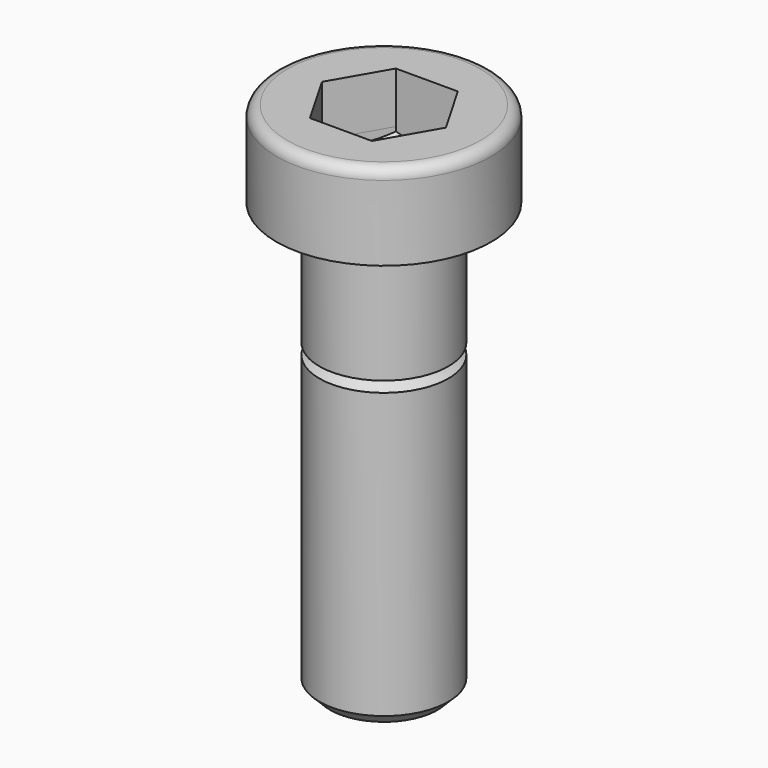
from build123d import *

# Parameters (mm, degrees)
F2_R     = 0.5
F3_SIZE  = 0.5
F5_DEPTH = 2.38


# Not quite as in the source:
# - a fillet or chamfer that OpenCascade refuses, or shapes differently, is made with other operations: its cross-section is extruded or revolved along the edge and cut away or added


with BuildPart() as f1:
    # F0 (on Front) → F1 (revolve)
    with BuildSketch(Plane.XZ):
        Polygon((-3, 0), (0, 0), (0, 18), (-1.5, 18.8660254038), (-1.5, 24), (-5, 24), (-5, 20), (-3, 20), (-3, 14.25), (-2.5, 14), (-3, 13.75), align=None)
    revolve(axis=Axis((0, 0, 18.332445994), (0, 0, 1)))

    # F2
    f2_edges = [f1.edges().sort_by_distance(p)[0] for p in [
        (5, 0, 24),
    ]]
    fillet(f2_edges, radius=F2_R)

    # F3
    f3_edges = [f1.edges().sort_by_distance(p)[0] for p in [
        (3, 0, 0),
    ]]
    chamfer(f3_edges, length=F3_SIZE)

    # F4 (on face) → F5 (cut)
    with BuildSketch(Plane.XY.offset(24)):
        Polygon((-1.443375673, -2.5), (1.443375673, -2.5), (2.8867513459, 0), (1.443375673, 2.5), (-1.443375673, 2.5), (-2.8867513459, 0), align=None)
    extrude(amount=-F5_DEPTH, mode=Mode.SUBTRACT)

    # F6: chamfer of 1 x 1.7320508076 on 1 edges, made by hand


with BuildPart() as f6_tool2:
    # F6_s3 → F6_t4 (revolve)
    with BuildSketch(Plane.XZ):
        Polygon((-3.2320508076, 21.62), (-1.5, 20.62), (-1.5, 21.62), align=None)
    revolve(axis=Axis((0, 0, 21.62), (0, 0, 1)))

    split(bisect_by=Plane(origin=(-2.1650635095, 1.25, 0), x_dir=(0, 0, 1), z_dir=(0.8660254038, -0.5, 0)), keep=Keep.TOP)

    split(bisect_by=Plane.XZ.offset(-2.5), keep=Keep.TOP)

    split(bisect_by=Plane(origin=(2.1650635095, 1.25, 0), x_dir=(0, 0, 1), z_dir=(-0.8660254038, -0.5, 0)), keep=Keep.TOP)

    split(bisect_by=Plane(origin=(2.1650635095, -1.25, 0), x_dir=(0, 0, 1), z_dir=(-0.8660254038, 0.5, 0)), keep=Keep.TOP)

    split(bisect_by=Plane.XZ.offset(2.5), keep=Keep.BOTTOM)

    split(bisect_by=Plane(origin=(-2.1650635095, -1.25, 0), x_dir=(0, 0, 1), z_dir=(0.8660254038, 0.5, 0)), keep=Keep.TOP)


with BuildPart() as f1_1:
    add(f1.part)

    # F6_t1: cut F6_tool2
    add(f6_tool2.part, mode=Mode.SUBTRACT)


solid = f1_1.part
